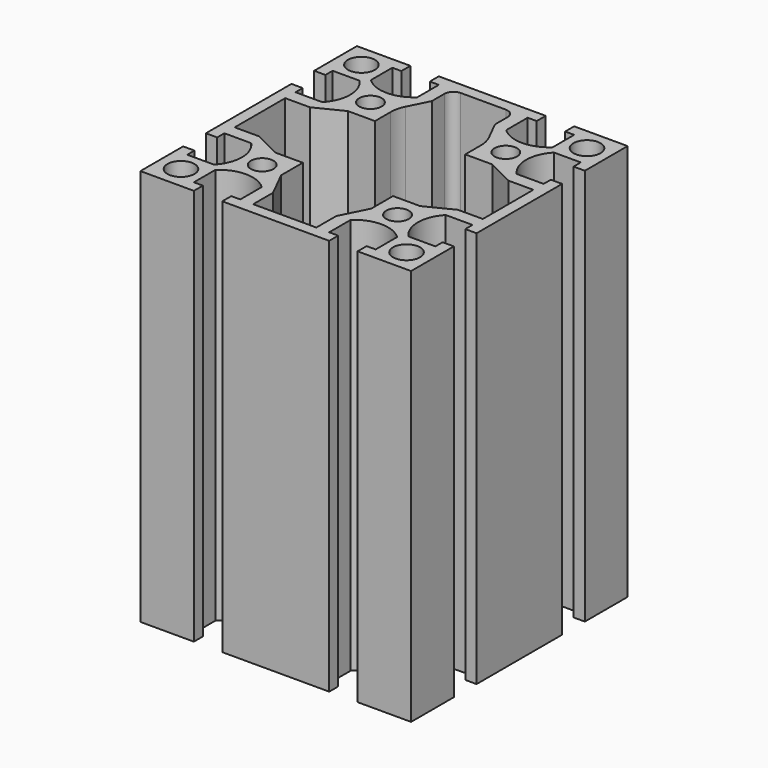
from build123d import *

# Parameters (mm, degrees)
F0_R     = 3
F0_R_2   = 2.5
F1_DEPTH = 87.98
F2_R     = 2
F3_R     = 7


# Not quite as in the source:
# - a feature names something its author has since deleted; it is built from what else it names


with BuildPart() as f1:
    # F0 (on Top) → F1 (new body)
    with BuildSketch(Plane.XY):
        with BuildLine():
            Line((18.15, -30), (30, -30))
            Line((30, -30), (30, -18.15))
            Line((30, -18.15), (27.5, -18.15))
            Line((27.5, -18.15), (27.5, -20.15))
            Line((27.5, -20.15), (21.5477069044, -20.15))
            ThreePointArc((21.5477069044, -20.15), (19.5, -15), (21.5477069044, -9.85))
            Line((21.5477069044, -9.85), (27.5, -9.85))
            Line((27.5, -9.85), (27.5, -11.85))
            Line((27.5, -11.85), (30, -11.85))
            Line((30, -11.85), (30, 11.85))
            Line((30, 11.85), (27.5, 11.85))
            Line((27.5, 11.85), (27.5, 9.85))
            Line((27.5, 9.85), (21.5477069044, 9.85))
            ThreePointArc((21.5477069044, 9.85), (19.5, 15), (21.5477069044, 20.15))
            Line((21.5477069044, 20.15), (27.5, 20.15))
            Line((27.5, 20.15), (27.5, 18.15))
            Line((27.5, 18.15), (30, 18.15))
            Line((30, 18.15), (30, 30))
            Line((30, 30), (18.15, 30))
            Line((18.15, 30), (18.15, 27.5))
            Line((18.15, 27.5), (20.15, 27.5))
            Line((20.15, 27.5), (20.15, 21.5477069044))
            ThreePointArc((20.15, 21.5477069044), (15, 19.5), (9.85, 21.5477069044))
            Line((9.85, 21.5477069044), (9.85, 27.5))
            Line((9.85, 27.5), (11.85, 27.5))
            Line((11.85, 27.5), (11.85, 30))
            Line((11.85, 30), (-11.85, 30))
            Line((-11.85, 30), (-11.85, 27.5))
            Line((-11.85, 27.5), (-9.85, 27.5))
            Line((-9.85, 27.5), (-9.85, 21.5477069044))
            ThreePointArc((-9.85, 21.5477069044), (-15, 19.5), (-20.15, 21.5477069044))
            Line((-20.15, 21.5477069044), (-20.15, 27.5))
            Line((-20.15, 27.5), (-18.15, 27.5))
            Line((-18.15, 27.5), (-18.15, 30))
            Line((-18.15, 30), (-30, 30))
            Line((-30, 30), (-30, 18.15))
            Line((-30, 18.15), (-27.5, 18.15))
            Line((-27.5, 18.15), (-27.5, 20.15))
            Line((-27.5, 20.15), (-21.5477069044, 20.15))
            ThreePointArc((-21.5477069044, 20.15), (-19.5, 15), (-21.5477069044, 9.85))
            Line((-21.5477069044, 9.85), (-27.5, 9.85))
            Line((-27.5, 9.85), (-27.5, 11.85))
            Line((-27.5, 11.85), (-30, 11.85))
            Line((-30, 11.85), (-30, -11.85))
            Line((-30, -11.85), (-27.5, -11.85))
            Line((-27.5, -11.85), (-27.5, -9.85))
            Line((-27.5, -9.85), (-21.5477069044, -9.85))
            ThreePointArc((-21.5477069044, -9.85), (-19.5, -15), (-21.5477069044, -20.15))
            Line((-21.5477069044, -20.15), (-27.5, -20.15))
            Line((-27.5, -20.15), (-27.5, -18.15))
            Line((-27.5, -18.15), (-30, -18.15))
            Line((-30, -18.15), (-30, -30))
            Line((-30, -30), (-18.15, -30))
            Line((-18.15, -30), (-18.15, -27.5))
            Line((-18.15, -27.5), (-20.15, -27.5))
            Line((-20.15, -27.5), (-20.15, -21.5477069044))
            ThreePointArc((-20.15, -21.5477069044), (-15, -19.5), (-9.85, -21.5477069044))
            Line((-9.85, -21.5477069044), (-9.85, -27.5))
            Line((-9.85, -27.5), (-11.85, -27.5))
            Line((-11.85, -27.5), (-11.85, -30))
            Line((-11.85, -30), (11.85, -30))
            Line((11.85, -30), (11.85, -27.5))
            Line((11.85, -27.5), (9.85, -27.5))
            Line((9.85, -27.5), (9.85, -21.5477069044))
            ThreePointArc((9.85, -21.5477069044), (15, -19.5), (20.15, -21.5477069044))
            Line((20.15, -21.5477069044), (20.15, -27.5))
            Line((20.15, -27.5), (18.15, -27.5))
            Line((18.15, -27.5), (18.15, -30))
        make_face()
        with Locations((-25, -25)):
            Circle(F0_R, mode=Mode.SUBTRACT)
        with Locations((-15, -15)):
            Circle(F0_R_2, mode=Mode.SUBTRACT)
        with Locations((25, -25)):
            Circle(F0_R, mode=Mode.SUBTRACT)
        with Locations((15, -15)):
            Circle(F0_R_2, mode=Mode.SUBTRACT)
        with Locations((-25, 25)):
            Circle(F0_R, mode=Mode.SUBTRACT)
        with Locations((-15, 15)):
            Circle(F0_R_2, mode=Mode.SUBTRACT)
        Polygon((-7, 22), (-7, 27.5), (0, 27.5), (7, 27.5), (7, 22), (10, 16), (10, 10), (16, 10), (22, 7), (27.5, 7), (27.5, 0), (27.5, -7), (22, -7), (16, -10), (10, -10), (10, -16), (7, -22), (7, -27.5), (0, -27.5), (-7, -27.5), (-7, -22), (-10, -16), (-10, -10), (-16, -10), (-22, -7), (-27.5, -7), (-27.5, 0), (-27.5, 7), (-22, 7), (-16, 10), (-10, 10), (-10, 16), align=None, mode=Mode.SUBTRACT)
        with Locations((15, 15)):
            Circle(F0_R_2, mode=Mode.SUBTRACT)
        with Locations((25, 25)):
            Circle(F0_R, mode=Mode.SUBTRACT)
    extrude(amount=F1_DEPTH)

    # F2
    f2_edges = [f1.edges().sort_by_distance(p)[0] for p in [
        (-7, 27.5, 43.99),
        (7, 27.5, 43.99),
    ]]
    fillet(f2_edges, radius=F2_R)

    # F3
    f3_edges = [f1.edges().sort_by_distance(p)[0] for p in [
        (-10, 16, 43.99),
        (10, 16, 43.99),
    ]]
    fillet(f3_edges, radius=F3_R)


solid = f1.part
